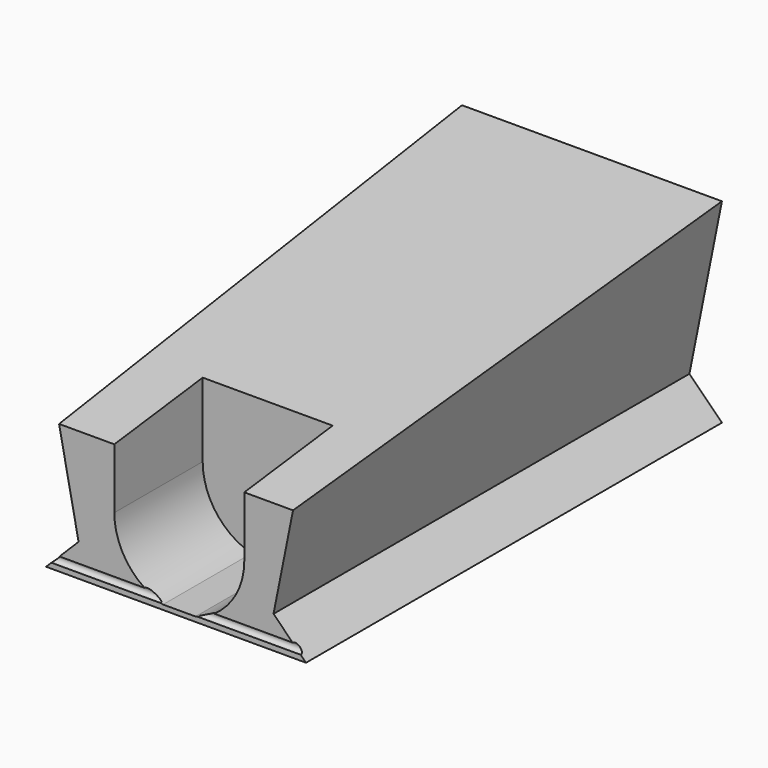
from build123d import *

# Parameters (mm, degrees)
F1_DEPTH = 101.6
F3_DEPTH = 50.8
F4_W     = 25.4
F4_H     = 7.2853491507
F5_DEPTH = 21.59
F7_R     = 0.79375
F8_DEPTH = 25.4


# Not quite as in the source:
# - a feature names something its author has since deleted; it is built from what else it names


with BuildPart() as f1:
    # F0 (on Front) → F1 (new body)
    with BuildSketch(Plane.XZ):
        Polygon((50.8, 31.75), (0, 31.75), (6.35, 0), (44.45, 0), align=None)
        Polygon((44.45, 0), (6.35, 0), (0, -6.35), (50.8, -6.35), align=None)
    extrude(amount=F1_DEPTH)

    # F2 (on Right) → F3 (cut)
    with BuildSketch(Plane.YZ):
        Polygon((-101.6, 31.75), (-101.6, 19.05), (0, 31.75), align=None)
    extrude(amount=F3_DEPTH, mode=Mode.SUBTRACT)

    # F4 (on face) → F5 (cut)
    with BuildSketch(Plane.XZ.offset(101.6)):
        with Locations((26.035, 22.6926745754)):
            Rectangle(F4_W, F4_H)
        with BuildLine():
            Line((13.335, 19.05), (13.335, 7.2853491507))
            ThreePointArc((13.335, 7.2853491507), (15.9808333333, -0.6521508493), (22.86, -5.4146508493))
            Line((22.86, -5.4146508493), (29.21, -5.4146508493))
            ThreePointArc((29.21, -5.4146508493), (36.0891666667, -0.6521508493), (38.735, 7.2853491507))
            Line((38.735, 7.2853491507), (38.735, 19.05))
            Line((38.735, 19.05), (13.335, 19.05))
        make_face()
    extrude(amount=-F5_DEPTH, mode=Mode.SUBTRACT)

    # F7 (on offset) → F8 (cut, symmetric)
    with BuildSketch(Plane.YZ.offset(26.035)):
        with Locations((-101.6, -4.5212)):
            Circle(F7_R)
    extrude(amount=F8_DEPTH, both=True, mode=Mode.SUBTRACT)


solid = f1.part
